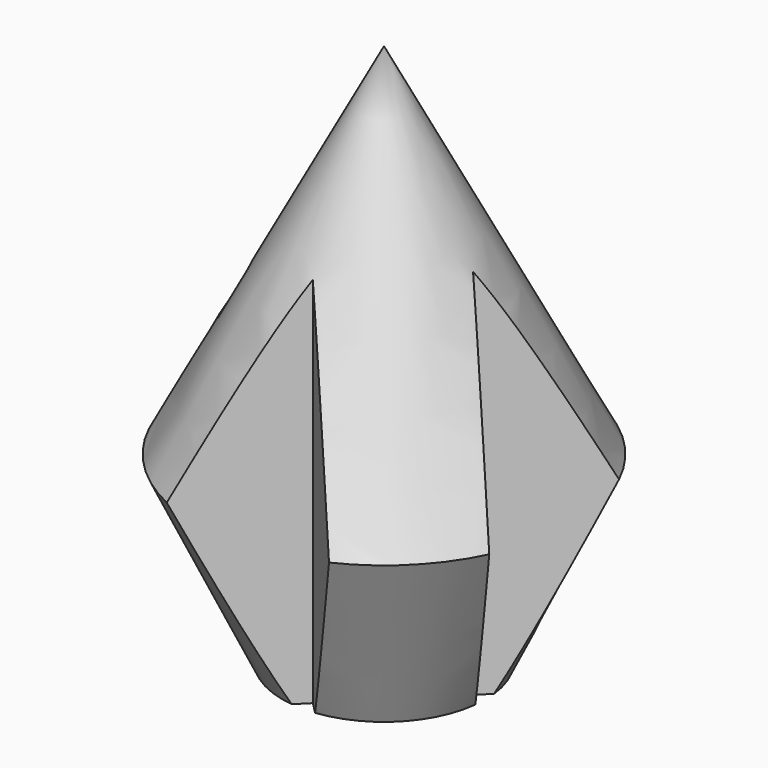
from build123d import *

# Parameters (mm, degrees)
F4_DEPTH = 26.7404350513


with BuildPart() as f1:
    # F0 (on Front) → F1 (revolve)
    with BuildSketch(Plane.XZ):
        Polygon((5, 0), (9.295072388, 9.0306341517), (0, 26.7394350513), (0, 0), align=None)
    revolve(axis=Axis((0, 0, -4.4079385259), (0, 0, -1)))

    # F3 (on face) → F4 (cut, through all)
    with BuildSketch(Plane.XY.offset(26.7394350513)):
        with BuildLine():
            ThreePointArc((9.295072388, 0), (9.0660769225, 2.0505169915), (8.3903736924, 4))
            Line((8.3903736924, 4), (4.3903736924, 0))
            Line((4.3903736924, 0), (8.3903736924, -4))
            ThreePointArc((8.3903736924, -4), (9.0660769225, -2.0505169915), (9.295072388, 0))
        make_face()
        with BuildLine():
            ThreePointArc((4, 8.3903736924), (0, 9.295072388), (-4, 8.3903736924))
            Line((-4, 8.3903736924), (0, 4.3903736924))
            Line((0, 4.3903736924), (4, 8.3903736924))
        make_face()
        with BuildLine():
            Line((-4.3903736924, 0), (-8.3903736924, 4))
            ThreePointArc((-8.3903736924, 4), (-9.295072388, 0), (-8.3903736924, -4))
            Line((-8.3903736924, -4), (-4.3903736924, 0))
        make_face()
        with BuildLine():
            Line((0, -4.3903736924), (-4, -8.3903736924))
            ThreePointArc((-4, -8.3903736924), (0, -9.295072388), (4, -8.3903736924))
            Line((4, -8.3903736924), (0, -4.3903736924))
        make_face()
    extrude(amount=-F4_DEPTH, mode=Mode.SUBTRACT)


solid = f1.part
